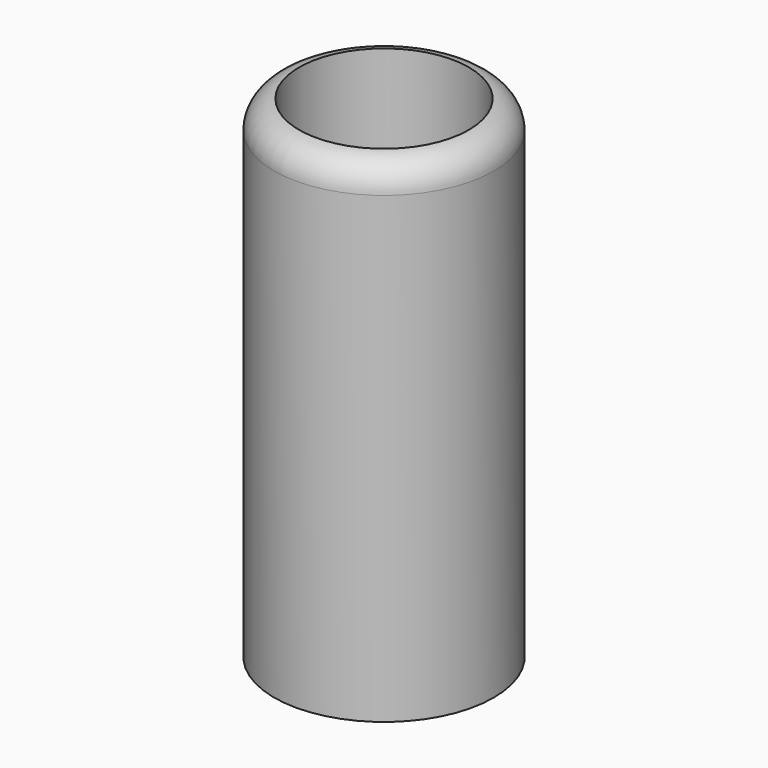
from build123d import *

# Parameters (mm, degrees)
F0_W     = 19.7259690613
F0_H     = 88.3059669286
F2_R     = 15.24
F3_DEPTH = 87.63


# Not quite as in the source:
# - a fillet or chamfer that OpenCascade refuses, or shapes differently, is made with other operations: its cross-section is extruded or revolved along the edge and cut away or added


with BuildPart() as f1:
    # F0 (on Front) → F1 (revolve)
    with BuildSketch(Plane.XZ):
        with Locations((9.8629845306, -15.7623393461)):
            Rectangle(F0_W, F0_H)
    revolve(axis=Axis((0, 0, 0), (0, 0, -1)))

    # F2 (on face) → F3 (cut)
    with BuildSketch(Plane.XY.offset(28.3906441182)):
        Circle(F2_R)
    extrude(amount=-F3_DEPTH, mode=Mode.SUBTRACT)

    # F4: fillet of radius 5.08 on 1 edges, made by hand

    # F4_s1 → F4_t2 (revolve, cut)
    with BuildSketch(Plane.XZ):
        with BuildLine():
            ThreePointArc((15.24, 28.3906441182), (18.4422881448, 26.7210487336), (19.7259690613, 23.345495236))
            Line((19.7259690613, 23.345495236), (19.7259690613, 28.3906441182))
            Line((19.7259690613, 28.3906441182), (15.24, 28.3906441182))
        make_face()
    revolve(axis=Axis((0, 0, 28.3906441182), (0, 0, -1)), mode=Mode.SUBTRACT)


solid = f1.part
